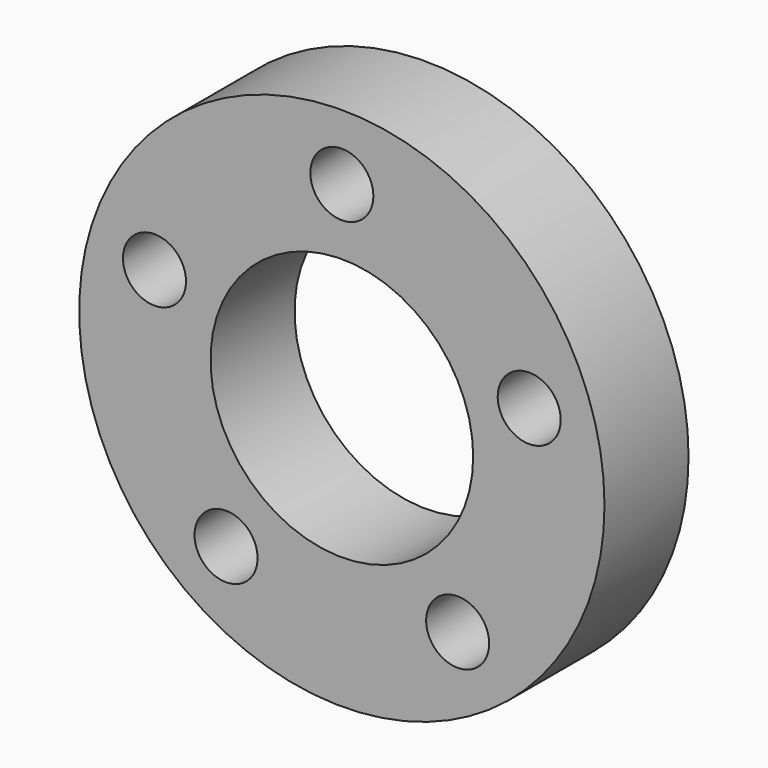
from build123d import *

# Parameters (mm, degrees)
F0_R            = 50
F0_R_2          = 25
F1_DEPTH        = 20
F2_R            = 6
F3_DEPTH        = 25
F3_COPIES_COUNT = 5


# Not quite as in the source:
# - a pattern or mirror of a feature is missing from the dataset's text; its kind, count and spacing are read off the source's solid


with BuildPart() as f1:
    # F0 (on Front) → F1 (new body)
    with BuildSketch(Plane.XZ):
        Circle(F0_R)
        Circle(F0_R_2, mode=Mode.SUBTRACT)
    extrude(amount=F1_DEPTH)

    # F2 (on face) → F3 (cut)
    with BuildSketch(Plane.XZ.offset(20)):
        with Locations((0, 37.5)):
            Circle(F2_R)
    f3 = extrude(amount=-F3_DEPTH, mode=Mode.SUBTRACT)

    # F3_copies: F3 ×5 about axis
    f3_copies_axis = Axis((0, 0, 0), (0, 1, 0))
    for i in range(1, F3_COPIES_COUNT):
        add(f3.rotate(f3_copies_axis, i * 360 / F3_COPIES_COUNT), mode=Mode.SUBTRACT)


solid = f1.part
